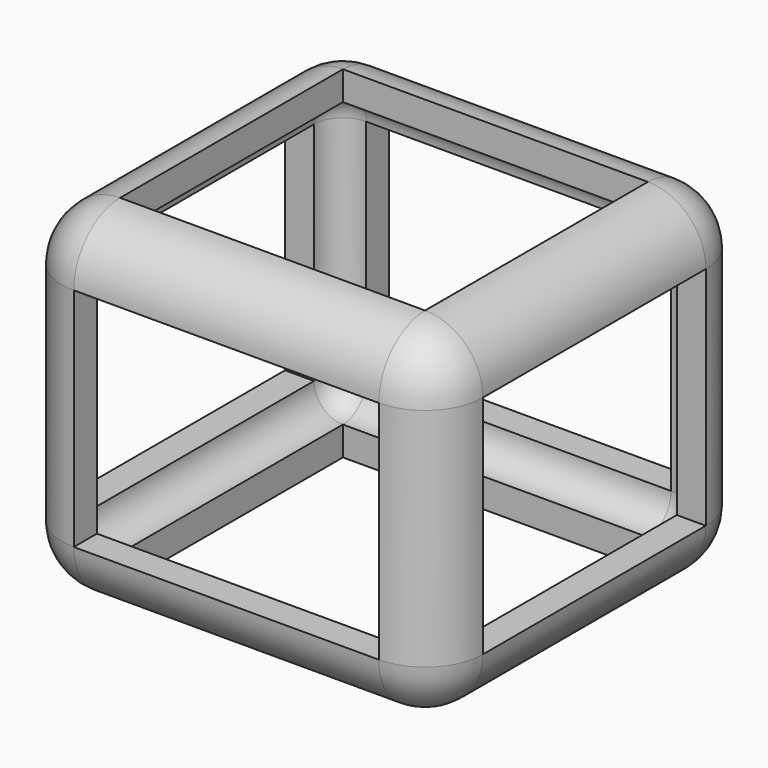
from build123d import *

# Parameters (mm, degrees)
F0_W     = 36.9340777397
F0_H     = 34.6101336181
F1_DEPTH = 30
F2_R     = 5.08
F3_T     = -2.54


# Not quite as in the source:
# - a shell that OpenCascade refuses in one call is made with other operations: the cavity is built on its own and cut out


with BuildPart() as f1:
    # F0 (on Top) → F1 (new body)
    with BuildSketch(Plane.XY):
        with Locations((18.4670388699, -17.3050668091)):
            Rectangle(F0_W, F0_H)
    extrude(amount=F1_DEPTH)

    # F2
    f2_edges = [f1.edges().sort_by_distance(p)[0] for p in [
        (36.934078, -34.610134, 15),
        (36.934078, 0, 15),
        (36.934078, -17.305067, 0),
        (18.467039, -34.610134, 0),
        (0, -17.305067, 0),
        (18.467039, 0, 0),
        (18.467039, 0, 30),
        (36.934078, -17.305067, 30),
        (18.467039, -34.610134, 30),
        (0, -34.610134, 15),
        (0, -17.305067, 30),
        (0, 0, 15),
    ]]
    fillet(f2_edges, radius=F2_R)

    # F3: a shell. OpenCascade refuses it in one call, so the cavity is built on its own and cut out:
    # the body offset inwards by the wall thickness, plus a prism from it out through each open face.
    f3_core = offset(f1.part, amount=F3_T, mode=Mode.PRIVATE)
    f3_exits = [f3_core.faces().sort_by_distance(p)[0] for p in [
        (18.467039, -17.305067, 27.46),
        (18.467039, -32.070134, 15),
        (18.467039, -2.54, 15),
        (2.54, -17.305067, 15),
        (18.467039, -17.305067, 2.54),
        (34.394078, -17.305067, 15),
    ]]
    add(f3_core, mode=Mode.SUBTRACT)
    extrude(f3_exits, amount=-F3_T, mode=Mode.SUBTRACT)


solid = f1.part
